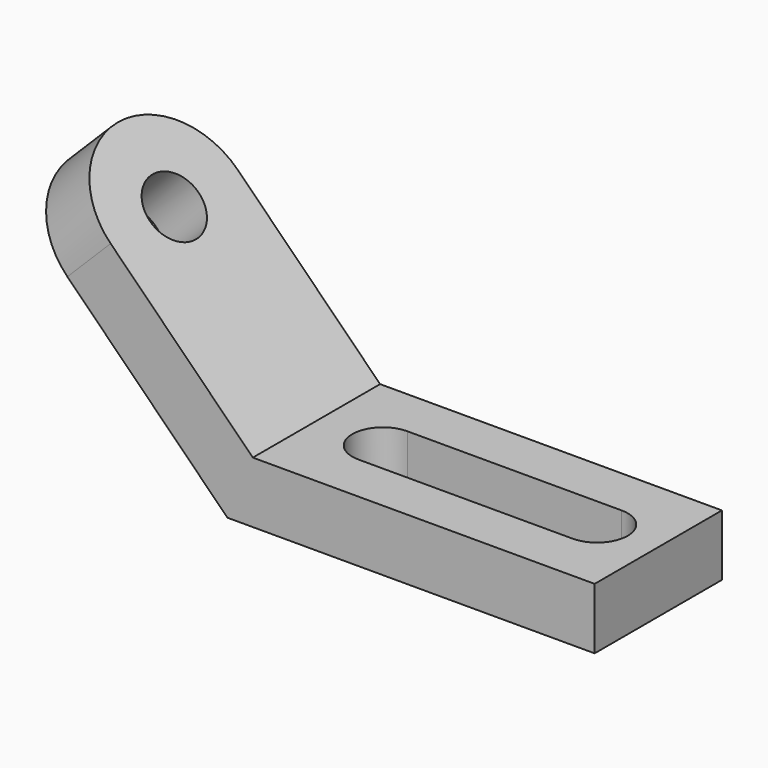
from build123d import *

# Parameters (mm, degrees)
F1_DEPTH = 52
F2_R     = 25.99999
F4_DEPTH = 26
F5_R     = 10
F6_DEPTH = 25


# Not quite as in the source:
# - a fillet or chamfer is up to 0.001 mm smaller than in the source, because OpenCascade refuses the exact size


with BuildPart() as f1:
    # F0 (on Front) → F1 (new body)
    with BuildSketch(Plane.XZ):
        Polygon((-156.8951708629, 103.594939314), (-86.1844927443, 32.8842611954), (33.8155072557, 32.8842611954), (33.8155072557, 52.8842611954), (-77.9002214968, 52.8842611954), (-142.7530352392, 117.7370749377), align=None)
    extrude(amount=F1_DEPTH)

    # F2 (radius 26 in the source; OpenCascade refuses exactly that, so slightly less here)
    f2_edges = [f1.edges().sort_by_distance(p)[0] for p in [
        (-149.824103, -52, 110.666007),
        (-149.824103, 0, 110.666007),
    ]]
    fillet(f2_edges, radius=F2_R)

    # F3 (on face) → F4 (cut)
    with BuildSketch(Plane(origin=(0, 0, 32.8842611954), x_dir=(1, 0, 0), z_dir=(0, 0, -1))):
        with BuildLine():
            ThreePointArc((-56.184492662, 36), (-66.1844927443, 26), (-56.184492662, 16))
            Line((-56.184492662, 16), (13.8155072557, 16))
            ThreePointArc((13.8155072557, 16), (23.8155072557, 26), (13.8155072557, 36))
            Line((13.8155072557, 36), (-56.184492662, 36))
        make_face()
    extrude(amount=-F4_DEPTH, mode=Mode.SUBTRACT)

    # F5 (on face) → F6 (cut)
    with BuildSketch(Plane(origin=(-12.5079801507, 0, -12.5079801507), x_dir=(0.7071067812, 0, -0.7071067812), z_dir=(0.7071067812, 0, 0.7071067812))):
        with Locations((-158.1943233382, -26)):
            Circle(F5_R)
    extrude(amount=-F6_DEPTH, mode=Mode.SUBTRACT)


solid = f1.part
